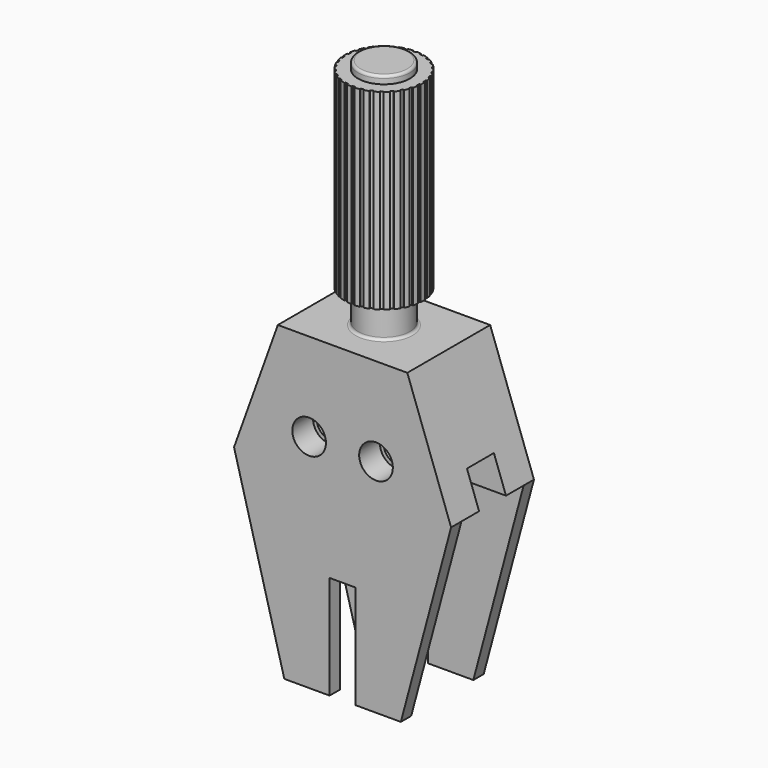
from build123d import *

# Parameters (mm, degrees)
F1_DEPTH         = 200
F2_R             = 100
F3_DEPTH         = 900
F5_R             = 150
F6_DEPTH         = 740
F8_DEPTH         = 580
F9_R             = 65
F9_R_2           = 50
F10_DEPTH        = 100
F11_DEPTH        = 350
F13_DEPTH        = 65
F14_R            = 10
F15_W            = 11.6287115961
F15_H            = 9.4758689404
F16_DEPTH        = 740
F16_COPIES_COUNT = 30


# Not quite as in the source:
# - a pattern or mirror of a feature is missing from the dataset's text; its kind, count and spacing are read off the source's solid


with BuildPart() as f1:
    # F0 (on Front) → F1 (new body, symmetric)
    with BuildSketch(Plane.XZ):
        Polygon((250, 794.9763654469), (-250, 794.9763654469), (-419.1142838269, 324.4443697168), (-225, -400), (-50, -400), (-50, 0), (0, 0), (50, 0), (50, -400), (225, -400), (419.1142838269, 324.4443697168), align=None)
    extrude(amount=F1_DEPTH, both=True)

    # F2 (on face) → F3 (join)
    with BuildSketch(Plane.XY.offset(794.9763654469)):
        Circle(F2_R)
    extrude(amount=F3_DEPTH)

    # F5 (on offset) → F6 (join)
    with BuildSketch(Plane.XY.offset(924.9763654469)):
        Circle(F5_R)
    extrude(amount=F6_DEPTH)

    # F7 (on Right) → F8 (cut, symmetric)
    with BuildSketch(Plane.YZ):
        Polygon((-150, 324.4443697168), (-150, -400), (150, -400), (150, 324.4443697168), (65, 324.4443697168), (65, 454.4443697168), (-65, 454.4443697168), (-65, 324.4443697168), align=None)
    extrude(amount=F8_DEPTH, both=True, mode=Mode.SUBTRACT)

    # F9 (on face) → F10 (cut)
    with BuildSketch(Plane.XZ.offset(200)):
        with Locations((-129.1142838269, 454.4443697168)):
            Circle(F9_R)
        with Locations((-129.1142838269, 454.4443697168)):
            Circle(F9_R_2, mode=Mode.SUBTRACT)
        with Locations((129.1142838269, 454.4443697168)):
            Circle(F9_R)
        with Locations((129.1142838269, 454.4443697168)):
            Circle(F9_R_2, mode=Mode.SUBTRACT)
    extrude(amount=-F10_DEPTH, mode=Mode.SUBTRACT)

    # F11 (cut): faces of the model
    f11_faces = [f1.faces().sort_by_distance(p)[0] for p in [
        (-129.1142838269, -200, 454.4443697168),
        (129.1142838269, -200, 454.4443697168),
    ]]
    extrude(f11_faces, amount=-F11_DEPTH, mode=Mode.SUBTRACT)

    # F12 (on Front) → F13 (cut, symmetric)
    with BuildSketch(Plane.XZ):
        Polygon((272.5361245925, 584.4443697168), (-272.5361245925, 584.4443697168), (-297.6948810114, 514.4443697168), (-372.3908790489, 454.4443697168), (-419.1142838269, 324.4443697168), (419.1142838269, 324.4443697168), (372.3908790489, 454.4443697168), (297.6948810114, 514.4443697168), align=None)
    extrude(amount=F13_DEPTH, both=True, mode=Mode.SUBTRACT)

    # F14
    f14_edges = [f1.edges().sort_by_distance(p)[0] for p in [
        (-100, 0, 1694.976365),
        (-100, 0, 794.976365),
    ]]
    fillet(f14_edges, radius=F14_R)

    # F15 (on face) → F16 (cut, through all)
    with BuildSketch(Plane.XY.offset(1664.9763654469)):
        with Locations((0, 150)):
            Rectangle(F15_W, F15_H)
    f16 = extrude(amount=-F16_DEPTH, mode=Mode.SUBTRACT)

    # F16_copies: F16 ×30 about axis
    f16_copies_axis = Axis((0, 0, 0), (0, 0, 1))
    for i in range(1, F16_COPIES_COUNT):
        add(f16.rotate(f16_copies_axis, i * 360 / F16_COPIES_COUNT), mode=Mode.SUBTRACT)


solid = f1.part
